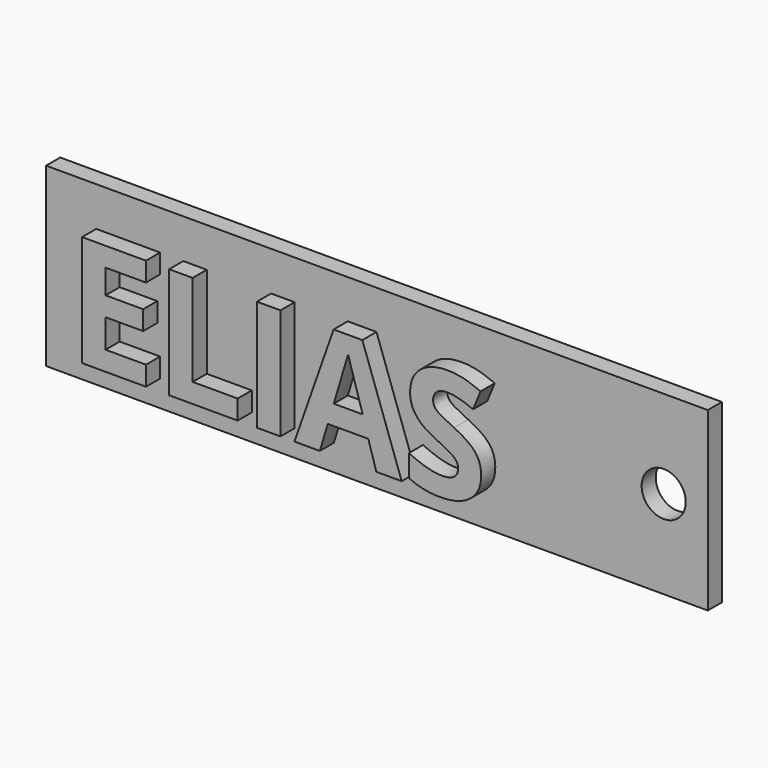
from build123d import *

# Parameters (mm, degrees)
F0_W         = 75
F0_H         = 20
F0_R         = 2.5
F2_DEPTH     = 2
F1_TEXT_SIZE = 12.1119968955
F3_DEPTH     = 2
F4_TEXT_SIZE = 17.6174501475
F5_DEPTH     = 2


# Not quite as in the source:
# - Text() gives the source's letters only with a copy of the font that has no kerning and outlines rounded to 1/6400 em; it was checked with that copy


with BuildPart() as f2:
    # F0 (on Front) → F2 (new body)
    with BuildSketch(Plane.XZ):
        with Locations((37.5, -10)):
            Rectangle(F0_W, F0_H)
        with Locations((70, -10)):
            Circle(F0_R, mode=Mode.SUBTRACT)
    extrude(amount=F2_DEPTH)

    # F1 (on face) → F3 (join)
    with BuildSketch(Plane.XZ):
        with Locations((6.8708048202, -14.4022656605)):
            Text('ELIAS', F1_TEXT_SIZE, font='Open Sans', font_style=FontStyle.BOLD, text_align=(TextAlign.LEFT, TextAlign.BOTTOM))
    extrude(amount=F3_DEPTH)

    # F4 (on face) → F5 (join)
    with BuildSketch(Plane.XZ.offset(2)):
        with Locations((4.0960581973, -17.0448832214)):
            Text('ELIAS', F4_TEXT_SIZE, font='Open Sans', font_style=FontStyle.BOLD, text_align=(TextAlign.LEFT, TextAlign.BOTTOM))
    extrude(amount=F5_DEPTH)


solid = f2.part
